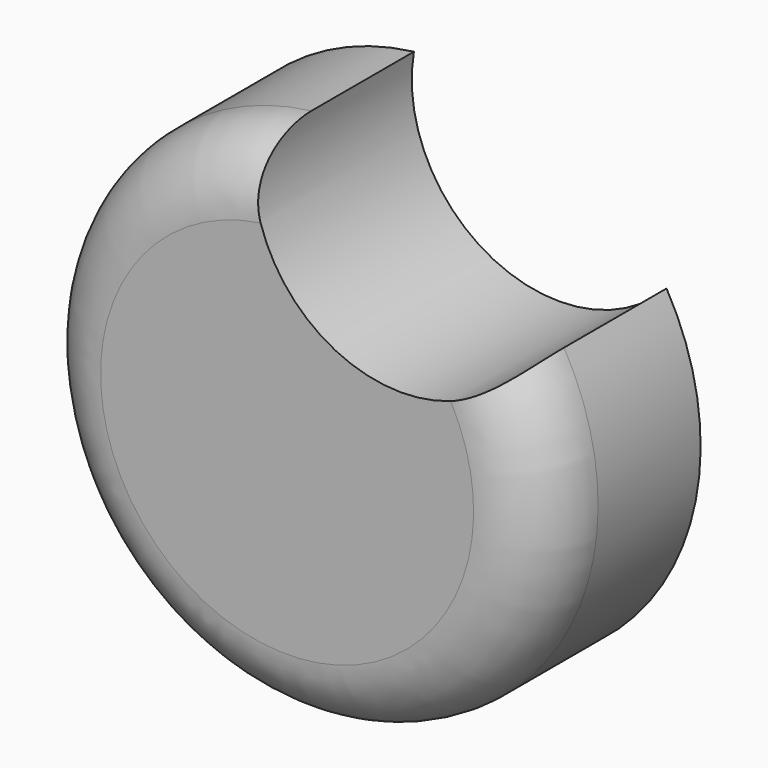
from build123d import *

# Parameters (mm, degrees)
F1_DEPTH = 31.496
F2_R     = 11.0377844072


# Not quite as in the source:
# - the program builds the solid bodies; features that only make, move or delete a surface that nothing else refers to are left out


with BuildPart() as f1:
    # F0 (on Front) → F1 (new body)
    with BuildSketch(Plane.XZ):
        with BuildLine():
            ThreePointArc((35.3676946952, 20.3558876834), (7.7172524441, 15.4458081316), (-4.959624117, 40.5047913221))
            ThreePointArc((-4.959624117, 40.5047913221), (-18.238894389, -36.5045027756), (35.3676946952, 20.3558876834))
        make_face()
    extrude(amount=F1_DEPTH)

    # F2
    f2_edges = [f1.edges().sort_by_distance(p)[0] for p in [
        (-18.238894, -31.496, -36.504503),
    ]]
    fillet(f2_edges, radius=F2_R)


solid = f1.part
